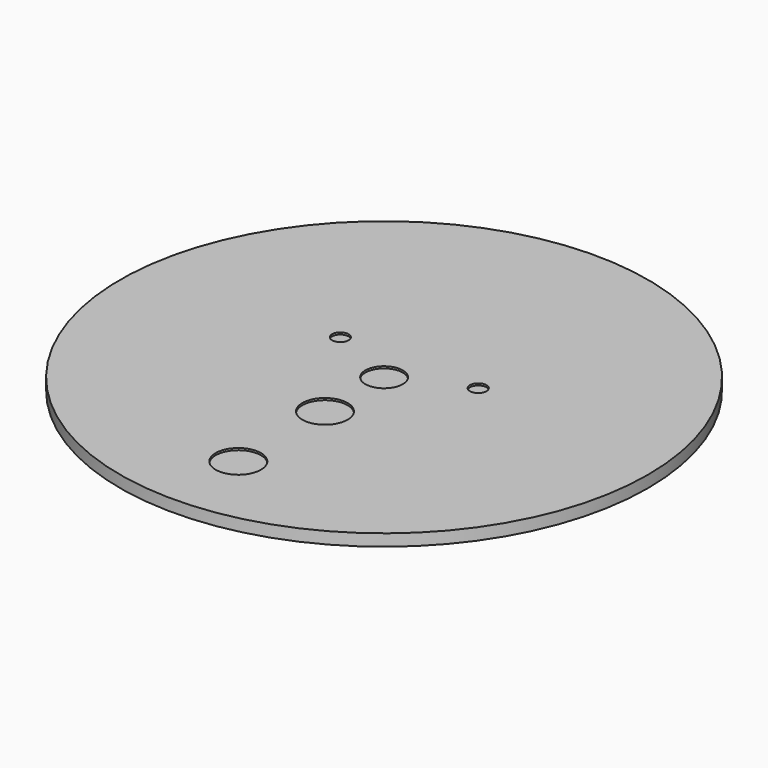
from build123d import *

# Parameters (mm, degrees)
F0_R     = 67
F1_DEPTH = 2.5
F4_DEPTH = 2
F6_R     = 2.1
F5_R     = 4.75
F5_R_2   = 5.75
F7_DEPTH = 0.501


# Not quite as in the source:
# - the program builds the solid bodies; features that only make, move or delete a surface that nothing else refers to are left out


with BuildPart() as f1:
    # F0 (on Top) → F1 (new body, symmetric)
    with BuildSketch(Plane.XY):
        Circle(F0_R)
    extrude(amount=F1_DEPTH, both=True)

    # F4 (cut): a face of the model
    f4_faces = [f1.faces().sort_by_distance(p)[0] for p in [
        (0, 0, 2.5),
    ]]
    extrude(f4_faces, amount=-F4_DEPTH, mode=Mode.SUBTRACT)

    # F6 (on Top) + F5 (on Top) → F7 (cut, through all)
    with BuildSketch(Plane.XY):
        with Locations((17.5, 8)):
            Circle(F6_R)
        with Locations((-17.5, 8)):
            Circle(F6_R)
    with BuildSketch(Plane.XY):
        Circle(F5_R)
        with Locations((0, -18.75)):
            Circle(F5_R_2)
        with Locations((0, -46.25)):
            Circle(F5_R_2)
    extrude(amount=F7_DEPTH, mode=Mode.SUBTRACT)


solid = f1.part
